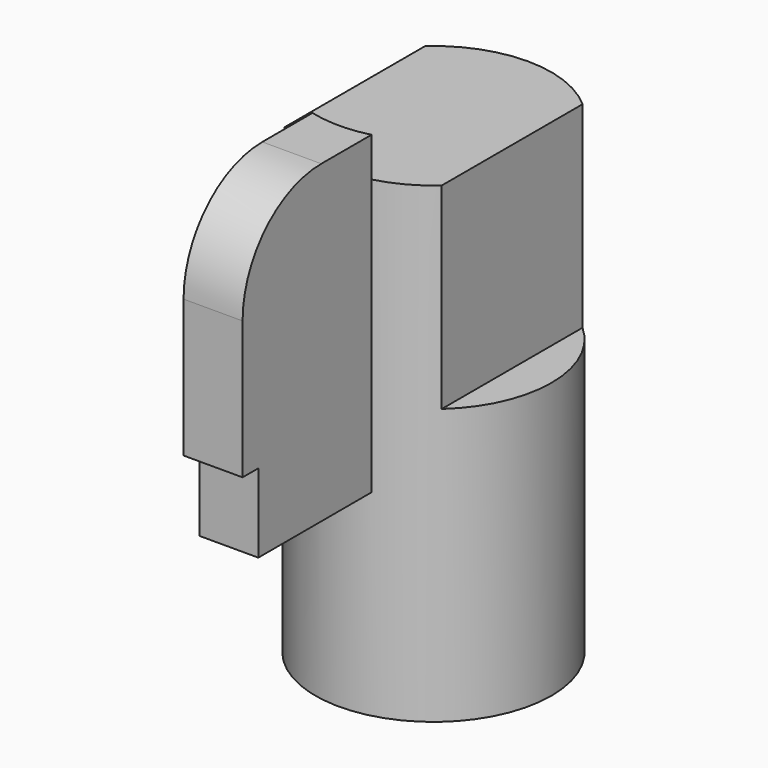
from build123d import *

# Parameters (mm, degrees)
F0_R      = 6
F1_DEPTH  = 10
F2_R      = 6
F3_DEPTH  = 6
F5_DEPTH  = 16
F7_DEPTH  = 8
F8_W      = 1
F8_H      = 4
F9_DEPTH  = 7.501
F10_DEPTH = 2


# Not quite as in the source:
# - a feature names something its author has since deleted; it is built from what else it names


with BuildPart() as f1:
    # F0 (on Top) → F1 (new body)
    with BuildSketch(Plane.XY):
        Circle(F0_R)
        with BuildLine():
            ThreePointArc((-2.1988001779, -1.9666666667), (0, 2.95), (2.1988001779, -1.9666666667))
            Line((2.1988001779, -1.9666666667), (-2.1988001779, -1.9666666667))
        make_face(mode=Mode.SUBTRACT)
    extrude(amount=F1_DEPTH)

    # F2 (on face) → F3 (join)
    with BuildSketch(Plane.XY.offset(10)):
        Circle(F2_R)
    extrude(amount=F3_DEPTH)



with BuildPart() as f5:
    # F4 (on face) → F5 (new body)
    with BuildSketch(Plane.XY.offset(10)):
        with BuildLine():
            ThreePointArc((1.5, -5.8094750193), (0, -6), (-1.5, -5.8094750193))
            Line((-1.5, -5.8094750193), (-1.5, -14))
            Line((-1.5, -14), (1.5, -14))
            Line((1.5, -14), (1.5, -5.8094750193))
        make_face()
    extrude(amount=F5_DEPTH)


with BuildPart() as f1_1:
    add(f1.part)

    add(f5.part)  # F7 merges F5
    # F6 (on face) → F7 (join)
    with BuildSketch(Plane.XY.offset(16)):
        with BuildLine():
            Line((-4, 4.472135955), (-4, -4.472135955))
            ThreePointArc((-4, -4.472135955), (0, -6), (4, -4.472135955))
            Line((4, -4.472135955), (4, 4.472135955))
            ThreePointArc((4, 4.472135955), (0, 6), (-4, 4.472135955))
        make_face()
    extrude(amount=F7_DEPTH)

    # F8 (on face) → F9 (cut, through all)
    with BuildSketch(Plane(origin=(-1.5, 0, 0), x_dir=(0, -1, 0), z_dir=(-1, 0, 0))):
        with BuildLine():
            ThreePointArc((9, 26), (12.5355339059, 24.5355339059), (14, 21))
            Line((14, 21), (14, 26))
            Line((14, 26), (9, 26))
        make_face()
        with Locations((13.5, 12)):
            Rectangle(F8_W, F8_H)
    extrude(amount=-F9_DEPTH, mode=Mode.SUBTRACT)

    # F6 (on face) → F10 (cut)
    with BuildSketch(Plane.XY.offset(16)):
        with BuildLine():
            Line((4, 4.472135955), (4, -4.472135955))
            ThreePointArc((4, -4.472135955), (5.4772255751, -2.4494897428), (6, 0))
            ThreePointArc((6, 0), (5.4772255751, 2.4494897428), (4, 4.472135955))
        make_face()
        with BuildLine():
            ThreePointArc((-4, 4.472135955), (-6, 0), (-4, -4.472135955))
            Line((-4, -4.472135955), (-4, 4.472135955))
        make_face()
    extrude(amount=-F10_DEPTH, mode=Mode.SUBTRACT)


solid = f1_1.part
